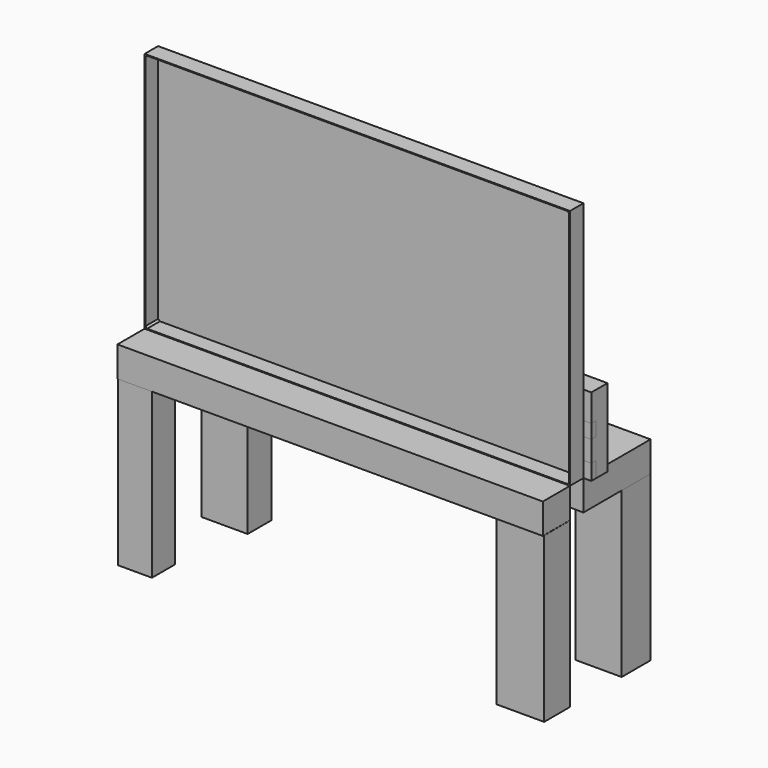
from build123d import *

# Parameters (mm, degrees)
F0_W      = 1282.7554736286
F0_H      = 729.6538352966
F1_DEPTH  = 50.8
F2_T      = -2.54
F3_SIZE   = 5.08
F4_W      = 1282.7554736286
F4_H      = 252.9141306877
F5_DEPTH  = 91.44
F4_H_2    = 102.3504243612
F6_W      = 102.859377861
F6_H      = 87.6475647092
F7_DEPTH  = 495.3
F6_W_2    = 139.9095300585
F6_H_2    = 108.8606417179
F6_W_3    = 139.4186019897
F6_H_3    = 89.6030068398
F6_W_4    = 143.9883280545
F6_H_4    = 98.3233042061
F8_W      = 207.591548562
F8_H      = 235.0982874632
F9_DEPTH  = 60.96
F8_W_2    = 201.7714977264
F10_W     = 44.2638136446
F10_H     = 42.4424037337
F11_DEPTH = 17.78
F10_W_2   = 55.2980303764
F10_H_2   = 41.7627468705
F10_H_3   = 47.184728086
F10_W_3   = 67.4202218652
F10_W_4   = 55.8717250824
F10_H_4   = 58.4349855781
F10_W_5   = 48.3711957932
F10_H_5   = 49.7663617134
F10_W_6   = 65.6886100769
F10_H_6   = 46.763850376
F10_W_7   = 31.4800739288
F10_H_7   = 37.3639315367


with BuildPart() as f1:
    # F0 (on Front) → F1 (new body)
    with BuildSketch(Plane.XZ):
        with Locations((-665.1519043371, 364.8269176483)):
            Rectangle(F0_W, F0_H)
    extrude(amount=F1_DEPTH)

    # F2
    f2_openings = [f1.faces().sort_by_distance(p)[0] for p in [
        (-665.151904, -50.8, 364.826918),
    ]]
    offset(amount=F2_T, openings=f2_openings)

    # F3
    f3_edges = [f1.edges().sort_by_distance(p)[0] for p in [
        (-1303.989641, -26.67, 727.113835),
        (-26.314168, -26.67, 727.113835),
        (-1303.989641, -26.67, 2.54),
        (-26.314168, -26.67, 2.54),
    ]]
    chamfer(f3_edges, length=F3_SIZE)


with BuildPart() as f5:
    # F4 (on face) → F5 (new body)
    with BuildSketch(Plane(origin=(0, 0, 0), x_dir=(1, 0, 0), z_dir=(0, 0, -1))):
        with Locations((-665.1519043371, -126.4570653439)):
            Rectangle(F4_W, F4_H)
    extrude(amount=F5_DEPTH)


with BuildPart() as f5b:
    # F4 (on face) → F5, piece 2 (new body)
    with BuildSketch(Plane(origin=(0, 0, 0), x_dir=(1, 0, 0), z_dir=(0, 0, -1))):
        with Locations((-665.1519043371, 101.9752121806)):
            Rectangle(F4_W, F4_H_2)
    extrude(amount=F5_DEPTH)


with BuildPart() as f7:
    # F6 (on face) → F7 (new body)
    with BuildSketch(Plane(origin=(0, 0, -91.44), x_dir=(1, 0, 0), z_dir=(0, 0, -1))):
        with Locations((-1255.0999522209, 107.9371087253)):
            Rectangle(F6_W, F6_H)
    extrude(amount=F7_DEPTH)


with BuildPart() as f7b:
    # F6 (on face) → F7, piece 2 (new body)
    with BuildSketch(Plane(origin=(0, 0, -91.44), x_dir=(1, 0, 0), z_dir=(0, 0, -1))):
        with Locations((-93.728932552, -198.4838098288)):
            Rectangle(F6_W_2, F6_H_2)
    extrude(amount=F7_DEPTH)


with BuildPart() as f7c:
    # F6 (on face) → F7, piece 3 (new body)
    with BuildSketch(Plane(origin=(0, 0, -91.44), x_dir=(1, 0, 0), z_dir=(0, 0, -1))):
        with Locations((-1236.8203401566, -208.1126272678)):
            Rectangle(F6_W_3, F6_H_3)
    extrude(amount=F7_DEPTH)


with BuildPart() as f7d:
    # F6 (on face) → F7, piece 4 (new body)
    with BuildSketch(Plane(origin=(0, 0, -91.44), x_dir=(1, 0, 0), z_dir=(0, 0, -1))):
        with Locations((-95.2921872959, 99.5689239353)):
            Rectangle(F6_W_4, F6_H_4)
    extrude(amount=F7_DEPTH)


with BuildPart() as f9:
    # F8 (on Front) → F9 (new body)
    with BuildSketch(Plane.XZ):
        with Locations((-103.795774281, 117.5491437316)):
            Rectangle(F8_W, F8_H)
    extrude(amount=-F9_DEPTH)


with BuildPart() as f9b:
    # F8 (on Front) → F9, piece 2 (new body)
    with BuildSketch(Plane.XZ):
        with Locations((-1209.2992067337, 117.5491437316)):
            Rectangle(F8_W_2, F8_H)
    extrude(amount=-F9_DEPTH)


with BuildPart() as f11:
    # F10 (on Front) → F11 (new body)
    with BuildSketch(Plane.XZ):
        with Locations((-22.1319068223, 131.5400190651)):
            Rectangle(F10_W, F10_H)
    extrude(amount=-F11_DEPTH)


with BuildPart() as f11b:
    # F10 (on Front) → F11, piece 2 (new body)
    with BuildSketch(Plane.XZ):
        with Locations((-130.7073384523, 131.2001906335)):
            Rectangle(F10_W_2, F10_H_2)
    extrude(amount=-F11_DEPTH)


with BuildPart() as f11c:
    # F10 (on Front) → F11, piece 3 (new body)
    with BuildSketch(Plane.XZ):
        with Locations((-22.1319068223, 23.592364043)):
            Rectangle(F10_W, F10_H_3)
    extrude(amount=-F11_DEPTH)


with BuildPart() as f11d:
    # F10 (on Front) → F11, piece 4 (new body)
    with BuildSketch(Plane.XZ):
        with Locations((-133.8455490768, 23.592364043)):
            Rectangle(F10_W_3, F10_H_3)
    extrude(amount=-F11_DEPTH)


with BuildPart() as f11e:
    # F10 (on Front) → F11, piece 5 (new body)
    with BuildSketch(Plane.XZ):
        with Locations((-1173.339009285, 125.806171447)):
            Rectangle(F10_W_4, F10_H_4)
    extrude(amount=-F11_DEPTH)


with BuildPart() as f11f:
    # F10 (on Front) → F11, piece 6 (new body)
    with BuildSketch(Plane.XZ):
        with Locations((-1256.7382454872, 105.3742915392)):
            Rectangle(F10_W_5, F10_H_5)
    extrude(amount=-F11_DEPTH)


with BuildPart() as f11g:
    # F10 (on Front) → F11, piece 7 (new body)
    with BuildSketch(Plane.XZ):
        with Locations((-1175.1223802567, 4.824702628)):
            Rectangle(F10_W_6, F10_H_6)
    extrude(amount=-F11_DEPTH)


with BuildPart() as f11h:
    # F10 (on Front) → F11, piece 8 (new body)
    with BuildSketch(Plane.XZ):
        with Locations((-1265.1838064194, 1.5210304409)):
            Rectangle(F10_W_7, F10_H_7)
    extrude(amount=-F11_DEPTH)


solid = Compound([f1.part, f5.part, f5b.part, f7.part, f7b.part, f7c.part, f7d.part, f9.part, f9b.part, f11.part, f11b.part, f11c.part, f11d.part, f11e.part, f11f.part, f11g.part, f11h.part])
